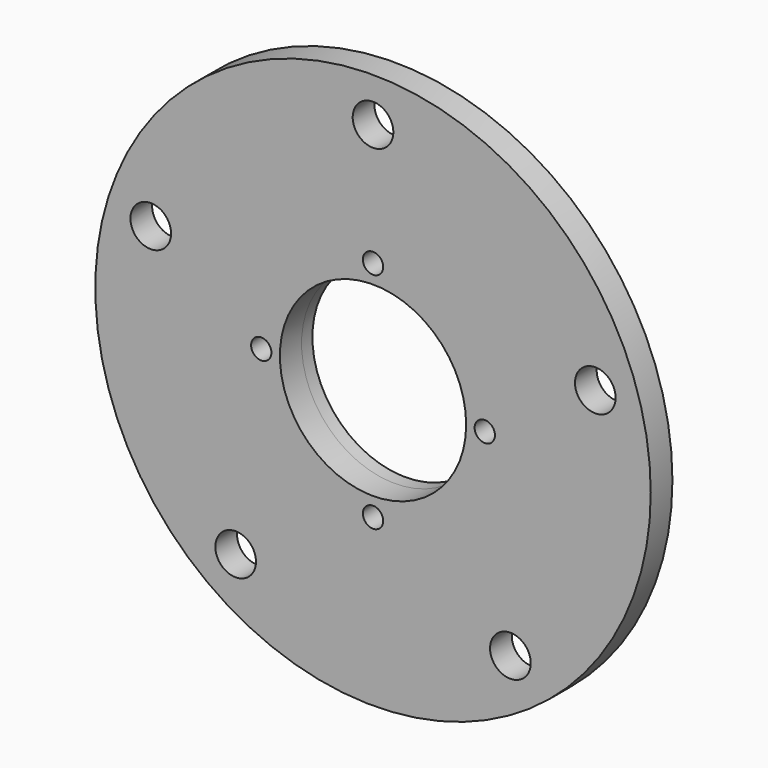
from build123d import *

# Parameters (mm, degrees)
F0_R            = 82
F0_R_2          = 56
F0_R_3          = 6
F0_R_4          = 27.5
F0_R_5          = 3
F1_DEPTH        = 8
F2_DEPTH        = 4
F3_DEPTH        = 8
F3_COPIES_COUNT = 5
F4_R            = 3
F5_DEPTH        = 12
F5_COPIES_COUNT = 4


# Not quite as in the source:
# - a pattern or mirror of a feature is missing from the dataset's text; its kind, count and spacing are read off the source's solid


with BuildPart() as f1:
    # F0 (on Front) → F1 (new body)
    with BuildSketch(Plane.XZ):
        Circle(F0_R)
        Circle(F0_R_2, mode=Mode.SUBTRACT)
        with Locations((0, 69)):
            Circle(F0_R_3, mode=Mode.SUBTRACT)
        Circle(F0_R_2)
        Circle(F0_R_4, mode=Mode.SUBTRACT)
        with Locations((0, 33)):
            Circle(F0_R_5, mode=Mode.SUBTRACT)
        with Locations((0, 69)):
            Circle(F0_R_3)
        with Locations((0, 33)):
            Circle(F0_R_5)
    extrude(amount=F1_DEPTH)

    # F0 (on Front) → F2 (join)
    with BuildSketch(Plane.XZ):
        Circle(F0_R_2)
        Circle(F0_R_4, mode=Mode.SUBTRACT)
        with Locations((0, 33)):
            Circle(F0_R_5, mode=Mode.SUBTRACT)
        with Locations((0, 33)):
            Circle(F0_R_5)
    extrude(amount=-F2_DEPTH)

    # F0 (on Front) → F3 (cut)
    with BuildSketch(Plane.XZ):
        with Locations((0, 69)):
            Circle(F0_R_3)
    f3 = extrude(amount=F3_DEPTH, mode=Mode.SUBTRACT)

    # F3_copies: F3 ×5 about axis
    f3_copies_axis = Axis((0, 0, 0), (0, 1, 0))
    for i in range(1, F3_COPIES_COUNT):
        add(f3.rotate(f3_copies_axis, i * 360 / F3_COPIES_COUNT), mode=Mode.SUBTRACT)

    # F4 (on face) → F5 (cut)
    with BuildSketch(Plane(origin=(0, 4, 0), x_dir=(-1, 0, 0), z_dir=(0, 1, 0))):
        with Locations((0, 33)):
            Circle(F4_R)
    f5 = extrude(amount=-F5_DEPTH, mode=Mode.SUBTRACT)

    # F5_copies: F5 ×4 about axis
    f5_copies_axis = Axis((0, 0, 0), (0, 1, 0))
    for i in range(1, F5_COPIES_COUNT):
        add(f5.rotate(f5_copies_axis, i * 360 / F5_COPIES_COUNT), mode=Mode.SUBTRACT)


solid = f1.part
